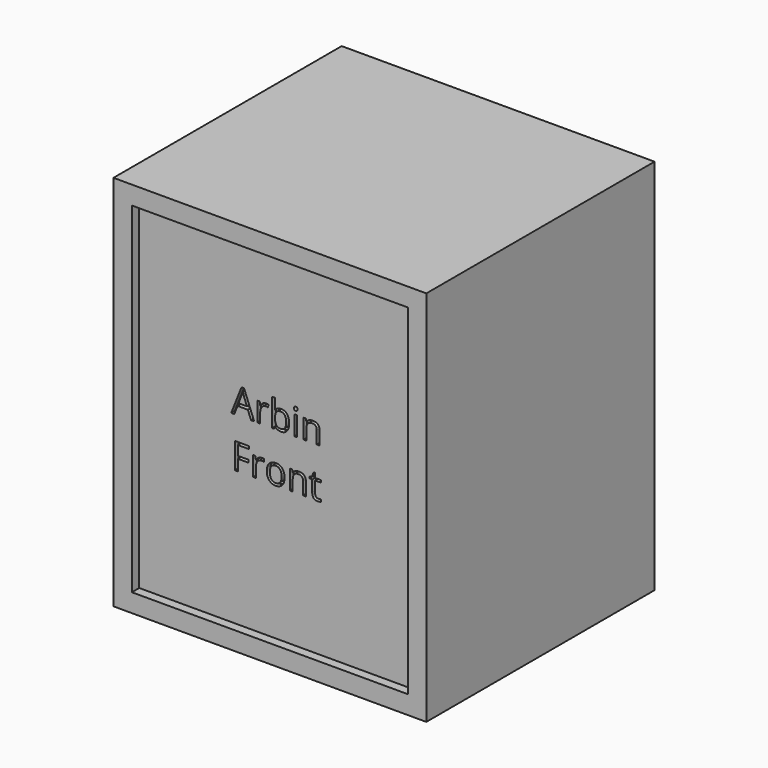
from build123d import *

# Parameters (mm, degrees)
F0_W         = 863.6
F0_H         = 787.4
F1_DEPTH     = 1041.4
F2_W         = 762
F2_H         = 939.8
F3_DEPTH     = 25.4
F4_TEXT_SIZE = 100.0369230769
F5_DEPTH     = 12.7


# Not quite as in the source:
# - Text() gives the source's letters only with a copy of the font that has no kerning and outlines rounded to 1/6400 em; it was checked with that copy


with BuildPart() as f1:
    # F0 (on Top) → F1 (new body)
    with BuildSketch(Plane.XY):
        Rectangle(F0_W, F0_H)
    extrude(amount=F1_DEPTH)

    # F2 (on face) → F3 (cut)
    with BuildSketch(Plane.XZ.offset(393.7)):
        with Locations((0, 520.7)):
            Rectangle(F2_W, F2_H)
    extrude(amount=-F3_DEPTH, mode=Mode.SUBTRACT)

    # F4 (on face) → F5 (cut)
    with BuildSketch(Plane.XZ.offset(368.3)):
        with Locations((-127, 558.8)):
            Text('Arbin', F4_TEXT_SIZE, font='Open Sans', text_align=(TextAlign.LEFT, TextAlign.BOTTOM))
        with Locations((-127, 422.7497846154)):
            Text('Front', F4_TEXT_SIZE, font='Open Sans', text_align=(TextAlign.LEFT, TextAlign.BOTTOM))
    extrude(amount=-F5_DEPTH, mode=Mode.SUBTRACT)


solid = f1.part
